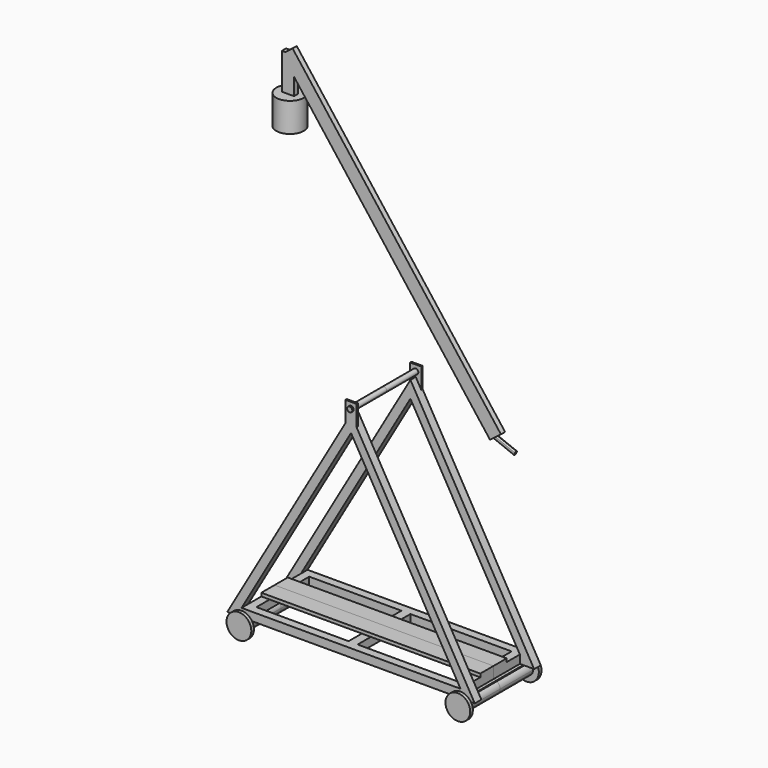
from build123d import *

# Parameters (mm, degrees)
F1_DEPTH       = 1.27
F2_W           = 1.2741235553
F2_H           = 1.2699995968
F2_W_2         = 1.3848708451
F2_W_3         = 1.2754402073
F3_DEPTH       = 5.08
F4_DEPTH       = 6.35
F6_DEPTH       = 0.508
F7_W           = 14.1913017724
F7_H           = 2.54
F7_W_2         = 1.2741235553
F7_W_3         = 1.3848708451
F7_W_4         = 15.5748559654
F7_W_5         = 1.2754402073
F8_DEPTH       = 0.508
F9_R           = 0.4024133142
F10_DEPTH      = 0.254
F11_DEPTH      = 0.254
F11_DEPTH_BACK = 6.35
F13_W          = 1.8706470204
F13_H          = 7.1249634751
F14_DEPTH      = 0.8
F15_R          = 2.114680679
F16_DEPTH      = 4.49
F18_START      = -0.2
F18_DEPTH      = 0.36
F19_T4_DEPTH   = 4.0914390002
F19_T9_DEPTH   = 4.0914390002
F19_T14_DEPTH  = 4.4938721404
F19_T19_DEPTH  = 4.4938721404


# Not quite as in the source:
# - a fillet or chamfer that OpenCascade refuses, or shapes differently, is made with other operations: its cross-section is extruded or revolved along the edge and cut away or added


with BuildPart() as f1:
    # F0 (on Front) → F1 (new body)
    with BuildSketch(Plane.XZ):
        Polygon((19.05, 32.9955678842), (0, 0), (1.6125002281, 0), (2.1992265269, 0), (2.8824598566, 0), (35.3591272308, 0), (35.8998188724, 0), (36.4111034397, 0), (38.1, 0), align=None)
        Polygon((35.9002961727, 1.2699995968), (2.1997038273, 1.2699995968), (19.05, 30.4555686905), align=None, mode=Mode.SUBTRACT)
    extrude(amount=F1_DEPTH)

    # F2 (on face) → F3 (join)
    with BuildSketch(Plane.XZ.offset(1.27)):
        with Locations((2.8367656049, 0.6349997984)):
            Rectangle(F2_W, F2_H)
        with Locations((18.3575645775, 0.6349997984)):
            Rectangle(F2_W_2, F2_H)
        with Locations((35.262576069, 0.6349997984)):
            Rectangle(F2_W_3, F2_H)
    extrude(amount=F3_DEPTH)

    # F0 (on Front) → F4 (join)
    with BuildSketch(Plane.XZ):
        with BuildLine():
            ThreePointArc((2.8824598566, -0.264036949), (2.5654652787, -0.0683053067), (2.1992265269, 0))
            ThreePointArc((2.1992265269, 0), (1.8913938178, -0.0477567136), (1.6125002281, -0.186537282))
            ThreePointArc((1.6125002281, -0.186537282), (1.7322454443, -1.9183226781), (3.2152269301, -1.0160004032))
            ThreePointArc((3.2152269301, -1.0160004032), (3.1283180611, -0.6048486789), (2.8824598566, -0.264036949))
        make_face()
        with BuildLine():
            ThreePointArc((36.4111034397, -0.138022664), (36.1646122657, -0.0351123983), (35.8998188724, 0))
            ThreePointArc((35.8998188724, 0), (35.6184705575, -0.0397320257), (35.3591272308, -0.1558205569))
            ThreePointArc((35.3591272308, -0.1558205569), (35.4084361837, -1.9052696945), (36.9158192755, -1.0160004032))
            ThreePointArc((36.9158192755, -1.0160004032), (36.7806486362, -0.5096450474), (36.4111034397, -0.138022664))
        make_face()
        with BuildLine():
            Line((2.1992265269, 0), (1.6125002281, 0))
            Line((1.6125002281, 0), (1.6125002281, -0.186537282))
            ThreePointArc((1.6125002281, -0.186537282), (1.8913938178, -0.0477567136), (2.1992265269, 0))
        make_face()
        with BuildLine():
            Line((36.4111034397, -0.138022664), (36.4111034397, 0))
            Line((36.4111034397, 0), (35.8998188724, 0))
            ThreePointArc((35.8998188724, 0), (36.1646122657, -0.0351123983), (36.4111034397, -0.138022664))
        make_face()
        with BuildLine():
            Line((35.8998188724, 0), (35.3591272308, 0))
            Line((35.3591272308, 0), (35.3591272308, -0.1558205569))
            ThreePointArc((35.3591272308, -0.1558205569), (35.6184705575, -0.0397320257), (35.8998188724, 0))
        make_face()
        with BuildLine():
            Line((2.8824598566, 0), (2.1992265269, 0))
            ThreePointArc((2.1992265269, 0), (2.5654652787, -0.0683053067), (2.8824598566, -0.264036949))
            Line((2.8824598566, -0.264036949), (2.8824598566, 0))
        make_face()
    extrude(amount=F4_DEPTH)

    # F5 (on face) → F6 (join)
    with BuildSketch(Plane(origin=(0, 0, 0), x_dir=(-1, 0, 0), z_dir=(0, 1, 0))):
        with BuildLine():
            Line((-35.3591272308, 0), (-34.2883697789, 0))
            ThreePointArc((-34.2883697789, 0), (-35.8998188724, 0.8889995968), (-37.5112679658, 0))
            Line((-37.5112679658, 0), (-36.4111034397, 0))
            Line((-36.4111034397, 0), (-36.4111034397, -0.138022664))
            ThreePointArc((-36.4111034397, -0.138022664), (-35.9170056479, -2.0318554293), (-35.3591272308, -0.1558205569))
            Line((-35.3591272308, -0.1558205569), (-35.3591272308, 0))
        make_face()
        with BuildLine():
            ThreePointArc((-37.5112679658, 0), (-36.4285978796, -2.8461418626), (-33.9948188724, -1.0160004032))
            ThreePointArc((-33.9948188724, -1.0160004032), (-34.0696774129, -0.4872213959), (-34.2883697789, 0))
            Line((-34.2883697789, 0), (-35.3591272308, 0))
            Line((-35.3591272308, 0), (-35.3591272308, -0.1558205569))
            ThreePointArc((-35.3591272308, -0.1558205569), (-35.9170056479, -2.0318554293), (-36.4111034397, -0.138022664))
            Line((-36.4111034397, -0.138022664), (-36.4111034397, 0))
            Line((-36.4111034397, 0), (-37.5112679658, 0))
        make_face()
        with BuildLine():
            Line((-2.8824598566, 0), (-3.8117017372, 0))
            ThreePointArc((-3.8117017372, 0), (-2.7279836056, -2.8470517609), (-0.293358451, -1.0160004032))
            ThreePointArc((-0.293358451, -1.0160004032), (-0.3681751692, -0.4872433245), (-0.5867513167, 0))
            Line((-0.5867513167, 0), (-1.6125002281, 0))
            Line((-1.6125002281, 0), (-1.6125002281, -0.186537282))
            ThreePointArc((-1.6125002281, -0.186537282), (-2.1373399263, -2.030114237), (-2.8824598566, -0.264036949))
            Line((-2.8824598566, -0.264036949), (-2.8824598566, 0))
        make_face()
        with BuildLine():
            ThreePointArc((-0.5867513167, 0), (-2.1992265269, 0.8898676727), (-3.8117017372, 0))
            Line((-3.8117017372, 0), (-2.8824598566, 0))
            Line((-2.8824598566, 0), (-2.8824598566, -0.264036949))
            ThreePointArc((-2.8824598566, -0.264036949), (-2.1373399263, -2.030114237), (-1.6125002281, -0.186537282))
            Line((-1.6125002281, -0.186537282), (-1.6125002281, 0))
            Line((-1.6125002281, 0), (-0.5867513167, 0))
        make_face()
    extrude(amount=F6_DEPTH)

    # F7 (on face) → F8 (join)
    with BuildSketch(Plane.XY.offset(1.2699995968)):
        with Locations((10.5694782687, -5.08)):
            Rectangle(F7_W, F7_H)
        with Locations((2.8367656049, -5.08)):
            Rectangle(F7_W_2, F7_H)
        with Locations((18.3575645775, -5.08)):
            Rectangle(F7_W_3, F7_H)
        with Locations((26.8374279827, -5.08)):
            Rectangle(F7_W_4, F7_H)
        with Locations((35.262576069, -5.08)):
            Rectangle(F7_W_5, F7_H)
    extrude(amount=F8_DEPTH)

    # F9 (on face) → F10 (join)
    with BuildSketch(Plane(origin=(0, 0, 0), x_dir=(-1, 0, 0), z_dir=(0, 1, 0))):
        Polygon((-19.9114145483, 34.6649885178), (-19.9114145483, 31.5035541202), (-19.05, 32.9955678842), (-18.1885854517, 31.5035541202), (-18.1885854517, 34.6649885178), align=None)
        with Locations((-19.05, 33.7386541069)):
            Circle(F9_R, mode=Mode.SUBTRACT)
        Polygon((-19.05, 32.9955678842), (-19.9114145483, 31.5035541202), (-18.1885854517, 31.5035541202), align=None)
    extrude(amount=-F10_DEPTH)

    # F9 (on face) → F11 (join, two sides)
    with BuildSketch(Plane(origin=(0, 0, 0), x_dir=(-1, 0, 0), z_dir=(0, 1, 0))) as f11_sk:
        with Locations((-19.05, 33.7386541069)):
            Circle(F9_R)
    extrude(amount=F11_DEPTH)
    extrude(f11_sk.sketch, amount=-F11_DEPTH_BACK)

    # F12: F1 across face


with BuildPart() as f1_1:
    add(f1.part)
    add(f1.part.mirror(Plane(origin=(18.9844198468, -6.35, 0.7885271629), x_dir=(1, 0, 0), z_dir=(0, -1, 0))))


with BuildPart() as f14:
    # F13 (on Front) → F14 (new body)
    with BuildSketch(Plane.XZ):
        Polygon((32.6115151858, 29.8361999529), (1.6799610114, 70.211231729), (0, 68.9242035151), (0.7575490221, 67.9353729614), (30.9315541743, 28.5491717389), align=None)
        Polygon((0, 68.9242035151), (1.6799610114, 70.211231729), (0.5408330401, 71.6981381993), (-0.5648436262, 70.851072669), (-1.1130979983, 70.4310517039), (-1.1130979983, 70.3771329992), align=None)
        Polygon((0.7575490221, 67.9353729614), (0, 68.9242035151), (-1.1130979983, 70.3771329992), (-1.1130979983, 67.9353729614), align=None)
        with Locations((-0.1777744881, 64.3728912239)):
            Rectangle(F13_W, F13_H)
        Polygon((-1.1130979983, 70.4310517039), (-0.5648436262, 70.851072669), (-1.1130979983, 70.851072669), align=None)
    extrude(amount=F14_DEPTH)

    # F15 (on face) → F16 (join)
    with BuildSketch(Plane(origin=(0, 0, 60.8104094863), x_dir=(1, 0, 0), z_dir=(0, 0, -1))):
        with Locations((-0.1777744881, 0.4)):
            Circle(F15_R)
        Polygon((0.7575490221, 0), (-0.1777744881, 0), (-1.1130979983, 0), (-1.1130979983, 0.8), (-0.1777744881, 0.8), (0.7575490221, 0.8), align=None, mode=Mode.SUBTRACT)
    extrude(amount=-F16_DEPTH)

    # F17 (on face) → F18 (join)
    with BuildSketch(Plane(origin=(0, 0, 0), x_dir=(-1, 0, 0), z_dir=(0, 1, 0)).offset(F18_START)):
        Polygon((-31.1495605422, 28.7161877258), (-31.77153468, 29.1926858459), (-34.645114094, 28.052713722), (-34.3972128675, 27.4278178617), align=None)
    extrude(amount=-F18_DEPTH)

    # F19: fillet of radius 0.2 on 4 edges, made by hand


with BuildPart() as f19_tool2:
    # F19_s3 → F19_t4 (new body)
    with BuildSketch(Plane(origin=(16.9803344824, 0, -6.7362356057), x_dir=(0, 1, 0), z_dir=(0.929528098, 0, -0.3687512915))):
        with BuildLine():
            ThreePointArc((-0.4, 38.8512161966), (-0.2585786438, 38.7926375529), (-0.2, 38.6512161966))
            Line((-0.2, 38.6512161966), (-0.2, 38.8512161966))
            Line((-0.2, 38.8512161966), (-0.4, 38.8512161966))
        make_face()
    extrude(amount=F19_T4_DEPTH)

    split(bisect_by=Plane(origin=(-2.3425232995, 0, 3.0577012755), x_dir=(0, 1, 0), z_dir=(0.6081511973, 0, -0.7938212149)), keep=Keep.TOP)


with BuildPart() as f14_1:
    add(f14.part)

    # F19_t1: cut F19_tool2
    add(f19_tool2.part, mode=Mode.SUBTRACT)


with BuildPart() as f19_tool7:
    # F19_s8 → F19_t9 (new body)
    with BuildSketch(Plane(origin=(16.9803344824, 0, -6.7362356057), x_dir=(0, 1, 0), z_dir=(0.929528098, 0, -0.3687512915))):
        with BuildLine():
            ThreePointArc((-0.56, 38.6512161966), (-0.5014213562, 38.7926375529), (-0.36, 38.8512161966))
            Line((-0.36, 38.8512161966), (-0.56, 38.8512161966))
            Line((-0.56, 38.8512161966), (-0.56, 38.6512161966))
        make_face()
    extrude(amount=F19_T9_DEPTH)

    split(bisect_by=Plane(origin=(-2.3425232995, 0, 3.0577012755), x_dir=(0, 1, 0), z_dir=(0.6081511973, 0, -0.7938212149)), keep=Keep.TOP)


with BuildPart() as f14_2:
    add(f14_1.part)

    # F19_t6: cut F19_tool7
    add(f19_tool7.part, mode=Mode.SUBTRACT)


with BuildPart() as f19_tool12:
    # F19_s13 → F19_t14 (new body)
    with BuildSketch(Plane(origin=(20.7834419944, 0, -8.244959021), x_dir=(0, 1, 0), z_dir=(-0.929528098, 0, 0.3687512915))):
        with BuildLine():
            ThreePointArc((-0.4, -38.1789440387), (-0.2585786438, -38.2375226825), (-0.2, -38.3789440387))
            Line((-0.2, -38.3789440387), (-0.2, -38.1789440387))
            Line((-0.2, -38.1789440387), (-0.4, -38.1789440387))
        make_face()
    extrude(amount=F19_T14_DEPTH)

    split(bisect_by=Plane(origin=(-2.3425232995, 0, 3.0577012755), x_dir=(0, 1, 0), z_dir=(0.6081511973, 0, -0.7938212149)), keep=Keep.TOP)


with BuildPart() as f14_3:
    add(f14_2.part)

    # F19_t11: cut F19_tool12
    add(f19_tool12.part, mode=Mode.SUBTRACT)


with BuildPart() as f19_tool17:
    # F19_s18 → F19_t19 (new body)
    with BuildSketch(Plane(origin=(20.7834419944, 0, -8.244959021), x_dir=(0, 1, 0), z_dir=(-0.929528098, 0, 0.3687512915))):
        with BuildLine():
            ThreePointArc((-0.36, -38.1789440387), (-0.5014213562, -38.2375226825), (-0.56, -38.3789440387))
            Line((-0.56, -38.3789440387), (-0.56, -38.1789440387))
            Line((-0.56, -38.1789440387), (-0.36, -38.1789440387))
        make_face()
    extrude(amount=F19_T19_DEPTH)

    split(bisect_by=Plane(origin=(-2.3425232995, 0, 3.0577012755), x_dir=(0, 1, 0), z_dir=(0.6081511973, 0, -0.7938212149)), keep=Keep.TOP)


with BuildPart() as f14_4:
    add(f14_3.part)

    # F19_t16: cut F19_tool17
    add(f19_tool17.part, mode=Mode.SUBTRACT)


solid = Compound([f1_1.part, f14_4.part])
